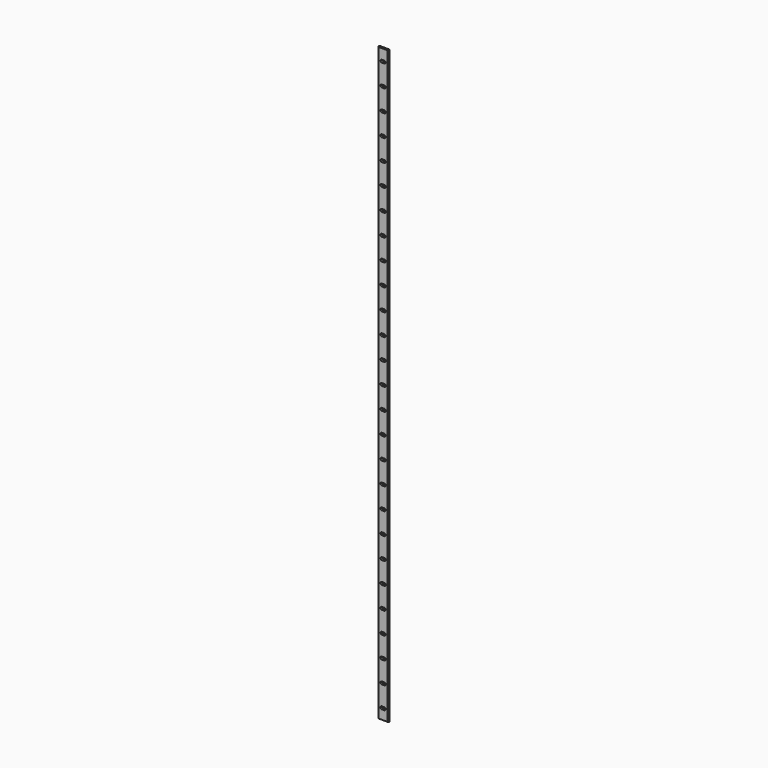
from build123d import *

# Parameters (mm, degrees)
F1_DEPTH = 1350
F2_R     = 0.5
F3_ANGLE = 180
F6_DEPTH = 25


with BuildPart() as f1:
    # F0 (on Top) → F1 (new body)
    with BuildSketch(Plane.XY):
        Polygon((20.122, 0), (0, 0), (0, -2.375), (19.5291, -2.375), (19.5291, -4.75), (20.122, -4.75), (22.497, -2.375), align=None)
    extrude(amount=F1_DEPTH)

    # F2
    f2_edges = [f1.edges().sort_by_distance(p)[0] for p in [
        (20.122, -4.75, 675),
        (22.497, -2.375, 675),
        (20.122, 0, 675),
    ]]
    fillet(f2_edges, radius=F2_R)


with BuildPart() as f3_1:
    # F3: copy of F1
    add(f1.part.rotate(Axis((0, -2.375, 675), (0, 0, -1)), F3_ANGLE))


with BuildPart() as f3_1_1:
    # F4: moved
    add(f3_1.part.moved(Location((19.5291, 0, 0))))


with BuildPart() as f6_tool:
    # F5 (on face) → F6 (new body)
    with BuildSketch(Plane.XZ.offset(4.75)):
        with BuildLine():
            ThreePointArc((6.7392067812, 1320.875), (8.4185023577, 1321.3645510123), (9.5716533906, 1322.6798215254))
            ThreePointArc((9.5716533906, 1322.6798215254), (10.7248044235, 1321.3645510123), (12.4041, 1320.875))
            ThreePointArc((12.4041, 1320.875), (15.5291, 1324), (12.4041, 1327.125))
            Line((12.4041, 1327.125), (6.7392067812, 1327.125))
            ThreePointArc((6.7392067812, 1327.125), (3.6142067812, 1324), (6.7392067812, 1320.875))
        make_face()
        with BuildLine():
            ThreePointArc((12.4041, 1320.875), (10.7248044235, 1321.3645510123), (9.5716533906, 1322.6798215254))
            ThreePointArc((9.5716533906, 1322.6798215254), (8.4185023577, 1321.3645510123), (6.7392067812, 1320.875))
            Line((6.7392067812, 1320.875), (12.4041, 1320.875))
        make_face()
        with BuildLine():
            Line((12.4041, 1277.125), (6.7392067812, 1277.125))
            ThreePointArc((6.7392067812, 1277.125), (3.6142067812, 1274), (6.7392067812, 1270.875))
            ThreePointArc((6.7392067812, 1270.875), (8.4185023577, 1271.3645510123), (9.5716533906, 1272.6798215254))
            ThreePointArc((9.5716533906, 1272.6798215254), (10.7248044235, 1271.3645510123), (12.4041, 1270.875))
            ThreePointArc((12.4041, 1270.875), (15.5291, 1274), (12.4041, 1277.125))
        make_face()
        with BuildLine():
            ThreePointArc((9.5716533906, 1272.6798215254), (8.4185023577, 1271.3645510123), (6.7392067812, 1270.875))
            Line((6.7392067812, 1270.875), (12.4041, 1270.875))
            ThreePointArc((12.4041, 1270.875), (10.7248044235, 1271.3645510123), (9.5716533906, 1272.6798215254))
        make_face()
        with BuildLine():
            Line((12.4041, 1227.125), (6.7392067812, 1227.125))
            ThreePointArc((6.7392067812, 1227.125), (3.6142067812, 1224), (6.7392067812, 1220.875))
            ThreePointArc((6.7392067812, 1220.875), (8.4185023577, 1221.3645510123), (9.5716533906, 1222.6798215254))
            ThreePointArc((9.5716533906, 1222.6798215254), (10.7248044235, 1221.3645510123), (12.4041, 1220.875))
            ThreePointArc((12.4041, 1220.875), (15.5291, 1224), (12.4041, 1227.125))
        make_face()
        with BuildLine():
            ThreePointArc((9.5716533906, 1222.6798215254), (8.4185023577, 1221.3645510123), (6.7392067812, 1220.875))
            Line((6.7392067812, 1220.875), (12.4041, 1220.875))
            ThreePointArc((12.4041, 1220.875), (10.7248044235, 1221.3645510123), (9.5716533906, 1222.6798215254))
        make_face()
        with BuildLine():
            Line((12.4041, 1177.125), (6.7392067812, 1177.125))
            ThreePointArc((6.7392067812, 1177.125), (3.6142067812, 1174), (6.7392067812, 1170.875))
            ThreePointArc((6.7392067812, 1170.875), (8.4185023577, 1171.3645510123), (9.5716533906, 1172.6798215254))
            ThreePointArc((9.5716533906, 1172.6798215254), (10.7248044235, 1171.3645510123), (12.4041, 1170.875))
            ThreePointArc((12.4041, 1170.875), (15.5291, 1174), (12.4041, 1177.125))
        make_face()
        with BuildLine():
            ThreePointArc((9.5716533906, 1172.6798215254), (8.4185023577, 1171.3645510123), (6.7392067812, 1170.875))
            Line((6.7392067812, 1170.875), (12.4041, 1170.875))
            ThreePointArc((12.4041, 1170.875), (10.7248044235, 1171.3645510123), (9.5716533906, 1172.6798215254))
        make_face()
        with BuildLine():
            Line((12.4041, 1127.125), (6.7392067812, 1127.125))
            ThreePointArc((6.7392067812, 1127.125), (3.6142067812, 1124), (6.7392067812, 1120.875))
            ThreePointArc((6.7392067812, 1120.875), (8.4185023577, 1121.3645510123), (9.5716533906, 1122.6798215254))
            ThreePointArc((9.5716533906, 1122.6798215254), (10.7248044235, 1121.3645510123), (12.4041, 1120.875))
            ThreePointArc((12.4041, 1120.875), (15.5291, 1124), (12.4041, 1127.125))
        make_face()
        with BuildLine():
            ThreePointArc((9.5716533906, 1122.6798215254), (8.4185023577, 1121.3645510123), (6.7392067812, 1120.875))
            Line((6.7392067812, 1120.875), (12.4041, 1120.875))
            ThreePointArc((12.4041, 1120.875), (10.7248044235, 1121.3645510123), (9.5716533906, 1122.6798215254))
        make_face()
        with BuildLine():
            Line((12.4041, 1077.125), (6.7392067812, 1077.125))
            ThreePointArc((6.7392067812, 1077.125), (3.6142067812, 1074), (6.7392067812, 1070.875))
            ThreePointArc((6.7392067812, 1070.875), (8.4185023577, 1071.3645510123), (9.5716533906, 1072.6798215254))
            ThreePointArc((9.5716533906, 1072.6798215254), (10.7248044235, 1071.3645510123), (12.4041, 1070.875))
            ThreePointArc((12.4041, 1070.875), (15.5291, 1074), (12.4041, 1077.125))
        make_face()
        with BuildLine():
            ThreePointArc((9.5716533906, 1072.6798215254), (8.4185023577, 1071.3645510123), (6.7392067812, 1070.875))
            Line((6.7392067812, 1070.875), (12.4041, 1070.875))
            ThreePointArc((12.4041, 1070.875), (10.7248044235, 1071.3645510123), (9.5716533906, 1072.6798215254))
        make_face()
        with BuildLine():
            Line((12.4041, 1027.125), (6.7392067812, 1027.125))
            ThreePointArc((6.7392067812, 1027.125), (3.6142067812, 1024), (6.7392067812, 1020.875))
            ThreePointArc((6.7392067812, 1020.875), (8.4185023577, 1021.3645510123), (9.5716533906, 1022.6798215254))
            ThreePointArc((9.5716533906, 1022.6798215254), (10.7248044235, 1021.3645510123), (12.4041, 1020.875))
            ThreePointArc((12.4041, 1020.875), (15.5291, 1024), (12.4041, 1027.125))
        make_face()
        with BuildLine():
            ThreePointArc((9.5716533906, 1022.6798215254), (8.4185023577, 1021.3645510123), (6.7392067812, 1020.875))
            Line((6.7392067812, 1020.875), (12.4041, 1020.875))
            ThreePointArc((12.4041, 1020.875), (10.7248044235, 1021.3645510123), (9.5716533906, 1022.6798215254))
        make_face()
        with BuildLine():
            Line((12.4041, 977.125), (6.7392067812, 977.125))
            ThreePointArc((6.7392067812, 977.125), (3.6142067812, 974), (6.7392067812, 970.875))
            ThreePointArc((6.7392067812, 970.875), (8.4185023577, 971.3645510123), (9.5716533906, 972.6798215254))
            ThreePointArc((9.5716533906, 972.6798215254), (10.7248044235, 971.3645510123), (12.4041, 970.875))
            ThreePointArc((12.4041, 970.875), (15.5291, 974), (12.4041, 977.125))
        make_face()
        with BuildLine():
            ThreePointArc((9.5716533906, 972.6798215254), (8.4185023577, 971.3645510123), (6.7392067812, 970.875))
            Line((6.7392067812, 970.875), (12.4041, 970.875))
            ThreePointArc((12.4041, 970.875), (10.7248044235, 971.3645510123), (9.5716533906, 972.6798215254))
        make_face()
        with BuildLine():
            Line((12.4041, 927.125), (6.7392067812, 927.125))
            ThreePointArc((6.7392067812, 927.125), (3.6142067812, 924), (6.7392067812, 920.875))
            ThreePointArc((6.7392067812, 920.875), (8.4185023577, 921.3645510123), (9.5716533906, 922.6798215254))
            ThreePointArc((9.5716533906, 922.6798215254), (10.7248044235, 921.3645510123), (12.4041, 920.875))
            ThreePointArc((12.4041, 920.875), (15.5291, 924), (12.4041, 927.125))
        make_face()
        with BuildLine():
            ThreePointArc((9.5716533906, 922.6798215254), (8.4185023577, 921.3645510123), (6.7392067812, 920.875))
            Line((6.7392067812, 920.875), (12.4041, 920.875))
            ThreePointArc((12.4041, 920.875), (10.7248044235, 921.3645510123), (9.5716533906, 922.6798215254))
        make_face()
        with BuildLine():
            Line((12.4041, 877.125), (6.7392067812, 877.125))
            ThreePointArc((6.7392067812, 877.125), (3.6142067812, 874), (6.7392067812, 870.875))
            ThreePointArc((6.7392067812, 870.875), (8.4185023577, 871.3645510123), (9.5716533906, 872.6798215254))
            ThreePointArc((9.5716533906, 872.6798215254), (10.7248044235, 871.3645510123), (12.4041, 870.875))
            ThreePointArc((12.4041, 870.875), (15.5291, 874), (12.4041, 877.125))
        make_face()
        with BuildLine():
            ThreePointArc((9.5716533906, 872.6798215254), (8.4185023577, 871.3645510123), (6.7392067812, 870.875))
            Line((6.7392067812, 870.875), (12.4041, 870.875))
            ThreePointArc((12.4041, 870.875), (10.7248044235, 871.3645510123), (9.5716533906, 872.6798215254))
        make_face()
        with BuildLine():
            Line((12.4041, 827.125), (6.7392067812, 827.125))
            ThreePointArc((6.7392067812, 827.125), (3.6142067812, 824), (6.7392067812, 820.875))
            ThreePointArc((6.7392067812, 820.875), (8.4185023577, 821.3645510123), (9.5716533906, 822.6798215254))
            ThreePointArc((9.5716533906, 822.6798215254), (10.7248044235, 821.3645510123), (12.4041, 820.875))
            ThreePointArc((12.4041, 820.875), (15.5291, 824), (12.4041, 827.125))
        make_face()
        with BuildLine():
            ThreePointArc((9.5716533906, 822.6798215254), (8.4185023577, 821.3645510123), (6.7392067812, 820.875))
            Line((6.7392067812, 820.875), (12.4041, 820.875))
            ThreePointArc((12.4041, 820.875), (10.7248044235, 821.3645510123), (9.5716533906, 822.6798215254))
        make_face()
        with BuildLine():
            Line((12.4041, 777.125), (6.7392067812, 777.125))
            ThreePointArc((6.7392067812, 777.125), (3.6142067812, 774), (6.7392067812, 770.875))
            ThreePointArc((6.7392067812, 770.875), (8.4185023577, 771.3645510123), (9.5716533906, 772.6798215254))
            ThreePointArc((9.5716533906, 772.6798215254), (10.7248044235, 771.3645510123), (12.4041, 770.875))
            ThreePointArc((12.4041, 770.875), (15.5291, 774), (12.4041, 777.125))
        make_face()
        with BuildLine():
            ThreePointArc((9.5716533906, 772.6798215254), (8.4185023577, 771.3645510123), (6.7392067812, 770.875))
            Line((6.7392067812, 770.875), (12.4041, 770.875))
            ThreePointArc((12.4041, 770.875), (10.7248044235, 771.3645510123), (9.5716533906, 772.6798215254))
        make_face()
        with BuildLine():
            Line((12.4041, 727.125), (6.7392067812, 727.125))
            ThreePointArc((6.7392067812, 727.125), (3.6142067812, 724), (6.7392067812, 720.875))
            ThreePointArc((6.7392067812, 720.875), (8.4185023577, 721.3645510123), (9.5716533906, 722.6798215254))
            ThreePointArc((9.5716533906, 722.6798215254), (10.7248044235, 721.3645510123), (12.4041, 720.875))
            ThreePointArc((12.4041, 720.875), (15.5291, 724), (12.4041, 727.125))
        make_face()
        with BuildLine():
            ThreePointArc((9.5716533906, 722.6798215254), (8.4185023577, 721.3645510123), (6.7392067812, 720.875))
            Line((6.7392067812, 720.875), (12.4041, 720.875))
            ThreePointArc((12.4041, 720.875), (10.7248044235, 721.3645510123), (9.5716533906, 722.6798215254))
        make_face()
        with BuildLine():
            Line((12.4041, 677.125), (6.7392067812, 677.125))
            ThreePointArc((6.7392067812, 677.125), (3.6142067812, 674), (6.7392067812, 670.875))
            ThreePointArc((6.7392067812, 670.875), (8.4185023577, 671.3645510123), (9.5716533906, 672.6798215254))
            ThreePointArc((9.5716533906, 672.6798215254), (10.7248044235, 671.3645510123), (12.4041, 670.875))
            ThreePointArc((12.4041, 670.875), (15.5291, 674), (12.4041, 677.125))
        make_face()
        with BuildLine():
            ThreePointArc((9.5716533906, 672.6798215254), (8.4185023577, 671.3645510123), (6.7392067812, 670.875))
            Line((6.7392067812, 670.875), (12.4041, 670.875))
            ThreePointArc((12.4041, 670.875), (10.7248044235, 671.3645510123), (9.5716533906, 672.6798215254))
        make_face()
        with BuildLine():
            Line((12.4041, 627.125), (6.7392067812, 627.125))
            ThreePointArc((6.7392067812, 627.125), (3.6142067812, 624), (6.7392067812, 620.875))
            ThreePointArc((6.7392067812, 620.875), (8.4185023577, 621.3645510123), (9.5716533906, 622.6798215254))
            ThreePointArc((9.5716533906, 622.6798215254), (10.7248044235, 621.3645510123), (12.4041, 620.875))
            ThreePointArc((12.4041, 620.875), (15.5291, 624), (12.4041, 627.125))
        make_face()
        with BuildLine():
            ThreePointArc((9.5716533906, 622.6798215254), (8.4185023577, 621.3645510123), (6.7392067812, 620.875))
            Line((6.7392067812, 620.875), (12.4041, 620.875))
            ThreePointArc((12.4041, 620.875), (10.7248044235, 621.3645510123), (9.5716533906, 622.6798215254))
        make_face()
        with BuildLine():
            Line((12.4041, 577.125), (6.7392067812, 577.125))
            ThreePointArc((6.7392067812, 577.125), (3.6142067812, 574), (6.7392067812, 570.875))
            ThreePointArc((6.7392067812, 570.875), (8.4185023577, 571.3645510123), (9.5716533906, 572.6798215254))
            ThreePointArc((9.5716533906, 572.6798215254), (10.7248044235, 571.3645510123), (12.4041, 570.875))
            ThreePointArc((12.4041, 570.875), (15.5291, 574), (12.4041, 577.125))
        make_face()
        with BuildLine():
            ThreePointArc((9.5716533906, 572.6798215254), (8.4185023577, 571.3645510123), (6.7392067812, 570.875))
            Line((6.7392067812, 570.875), (12.4041, 570.875))
            ThreePointArc((12.4041, 570.875), (10.7248044235, 571.3645510123), (9.5716533906, 572.6798215254))
        make_face()
        with BuildLine():
            Line((12.4041, 527.125), (6.7392067812, 527.125))
            ThreePointArc((6.7392067812, 527.125), (3.6142067812, 524), (6.7392067812, 520.875))
            ThreePointArc((6.7392067812, 520.875), (8.4185023577, 521.3645510123), (9.5716533906, 522.6798215254))
            ThreePointArc((9.5716533906, 522.6798215254), (10.7248044235, 521.3645510123), (12.4041, 520.875))
            ThreePointArc((12.4041, 520.875), (15.5291, 524), (12.4041, 527.125))
        make_face()
        with BuildLine():
            ThreePointArc((9.5716533906, 522.6798215254), (8.4185023577, 521.3645510123), (6.7392067812, 520.875))
            Line((6.7392067812, 520.875), (12.4041, 520.875))
            ThreePointArc((12.4041, 520.875), (10.7248044235, 521.3645510123), (9.5716533906, 522.6798215254))
        make_face()
        with BuildLine():
            Line((12.4041, 477.125), (6.7392067812, 477.125))
            ThreePointArc((6.7392067812, 477.125), (3.6142067812, 474), (6.7392067812, 470.875))
            ThreePointArc((6.7392067812, 470.875), (8.4185023577, 471.3645510123), (9.5716533906, 472.6798215254))
            ThreePointArc((9.5716533906, 472.6798215254), (10.7248044235, 471.3645510123), (12.4041, 470.875))
            ThreePointArc((12.4041, 470.875), (15.5291, 474), (12.4041, 477.125))
        make_face()
        with BuildLine():
            ThreePointArc((9.5716533906, 472.6798215254), (8.4185023577, 471.3645510123), (6.7392067812, 470.875))
            Line((6.7392067812, 470.875), (12.4041, 470.875))
            ThreePointArc((12.4041, 470.875), (10.7248044235, 471.3645510123), (9.5716533906, 472.6798215254))
        make_face()
        with BuildLine():
            Line((12.4041, 427.125), (6.7392067812, 427.125))
            ThreePointArc((6.7392067812, 427.125), (3.6142067812, 424), (6.7392067812, 420.875))
            ThreePointArc((6.7392067812, 420.875), (8.4185023577, 421.3645510123), (9.5716533906, 422.6798215254))
            ThreePointArc((9.5716533906, 422.6798215254), (10.7248044235, 421.3645510123), (12.4041, 420.875))
            ThreePointArc((12.4041, 420.875), (15.5291, 424), (12.4041, 427.125))
        make_face()
        with BuildLine():
            ThreePointArc((9.5716533906, 422.6798215254), (8.4185023577, 421.3645510123), (6.7392067812, 420.875))
            Line((6.7392067812, 420.875), (12.4041, 420.875))
            ThreePointArc((12.4041, 420.875), (10.7248044235, 421.3645510123), (9.5716533906, 422.6798215254))
        make_face()
        with BuildLine():
            Line((12.4041, 377.125), (6.7392067812, 377.125))
            ThreePointArc((6.7392067812, 377.125), (3.6142067812, 374), (6.7392067812, 370.875))
            ThreePointArc((6.7392067812, 370.875), (8.4185023577, 371.3645510123), (9.5716533906, 372.6798215254))
            ThreePointArc((9.5716533906, 372.6798215254), (10.7248044235, 371.3645510123), (12.4041, 370.875))
            ThreePointArc((12.4041, 370.875), (15.5291, 374), (12.4041, 377.125))
        make_face()
        with BuildLine():
            ThreePointArc((9.5716533906, 372.6798215254), (8.4185023577, 371.3645510123), (6.7392067812, 370.875))
            Line((6.7392067812, 370.875), (12.4041, 370.875))
            ThreePointArc((12.4041, 370.875), (10.7248044235, 371.3645510123), (9.5716533906, 372.6798215254))
        make_face()
        with BuildLine():
            Line((12.4041, 327.125), (6.7392067812, 327.125))
            ThreePointArc((6.7392067812, 327.125), (3.6142067812, 324), (6.7392067812, 320.875))
            ThreePointArc((6.7392067812, 320.875), (8.4185023577, 321.3645510123), (9.5716533906, 322.6798215254))
            ThreePointArc((9.5716533906, 322.6798215254), (10.7248044235, 321.3645510123), (12.4041, 320.875))
            ThreePointArc((12.4041, 320.875), (15.5291, 324), (12.4041, 327.125))
        make_face()
        with BuildLine():
            ThreePointArc((9.5716533906, 322.6798215254), (8.4185023577, 321.3645510123), (6.7392067812, 320.875))
            Line((6.7392067812, 320.875), (12.4041, 320.875))
            ThreePointArc((12.4041, 320.875), (10.7248044235, 321.3645510123), (9.5716533906, 322.6798215254))
        make_face()
        with BuildLine():
            Line((12.4041, 277.125), (6.7392067812, 277.125))
            ThreePointArc((6.7392067812, 277.125), (3.6142067812, 274), (6.7392067812, 270.875))
            ThreePointArc((6.7392067812, 270.875), (8.4185023577, 271.3645510123), (9.5716533906, 272.6798215254))
            ThreePointArc((9.5716533906, 272.6798215254), (10.7248044235, 271.3645510123), (12.4041, 270.875))
            ThreePointArc((12.4041, 270.875), (15.5291, 274), (12.4041, 277.125))
        make_face()
        with BuildLine():
            ThreePointArc((9.5716533906, 272.6798215254), (8.4185023577, 271.3645510123), (6.7392067812, 270.875))
            Line((6.7392067812, 270.875), (12.4041, 270.875))
            ThreePointArc((12.4041, 270.875), (10.7248044235, 271.3645510123), (9.5716533906, 272.6798215254))
        make_face()
        with BuildLine():
            Line((12.4041, 227.125), (6.7392067812, 227.125))
            ThreePointArc((6.7392067812, 227.125), (3.6142067812, 224), (6.7392067812, 220.875))
            ThreePointArc((6.7392067812, 220.875), (8.4185023577, 221.3645510123), (9.5716533906, 222.6798215254))
            ThreePointArc((9.5716533906, 222.6798215254), (10.7248044235, 221.3645510123), (12.4041, 220.875))
            ThreePointArc((12.4041, 220.875), (15.5291, 224), (12.4041, 227.125))
        make_face()
        with BuildLine():
            ThreePointArc((9.5716533906, 222.6798215254), (8.4185023577, 221.3645510123), (6.7392067812, 220.875))
            Line((6.7392067812, 220.875), (12.4041, 220.875))
            ThreePointArc((12.4041, 220.875), (10.7248044235, 221.3645510123), (9.5716533906, 222.6798215254))
        make_face()
        with BuildLine():
            Line((12.4041, 177.125), (6.7392067812, 177.125))
            ThreePointArc((6.7392067812, 177.125), (3.6142067812, 174), (6.7392067812, 170.875))
            ThreePointArc((6.7392067812, 170.875), (8.4185023577, 171.3645510123), (9.5716533906, 172.6798215254))
            ThreePointArc((9.5716533906, 172.6798215254), (10.7248044235, 171.3645510123), (12.4041, 170.875))
            ThreePointArc((12.4041, 170.875), (15.5291, 174), (12.4041, 177.125))
        make_face()
        with BuildLine():
            ThreePointArc((9.5716533906, 172.6798215254), (8.4185023577, 171.3645510123), (6.7392067812, 170.875))
            Line((6.7392067812, 170.875), (12.4041, 170.875))
            ThreePointArc((12.4041, 170.875), (10.7248044235, 171.3645510123), (9.5716533906, 172.6798215254))
        make_face()
        with BuildLine():
            Line((12.4041, 127.125), (6.7392067812, 127.125))
            ThreePointArc((6.7392067812, 127.125), (3.6142067812, 124), (6.7392067812, 120.875))
            ThreePointArc((6.7392067812, 120.875), (8.4185023577, 121.3645510123), (9.5716533906, 122.6798215254))
            ThreePointArc((9.5716533906, 122.6798215254), (10.7248044235, 121.3645510123), (12.4041, 120.875))
            ThreePointArc((12.4041, 120.875), (15.5291, 124), (12.4041, 127.125))
        make_face()
        with BuildLine():
            ThreePointArc((9.5716533906, 122.6798215254), (8.4185023577, 121.3645510123), (6.7392067812, 120.875))
            Line((6.7392067812, 120.875), (12.4041, 120.875))
            ThreePointArc((12.4041, 120.875), (10.7248044235, 121.3645510123), (9.5716533906, 122.6798215254))
        make_face()
        with BuildLine():
            Line((12.4041, 77.125), (6.7392067812, 77.125))
            ThreePointArc((6.7392067812, 77.125), (3.6142067812, 74), (6.7392067812, 70.875))
            ThreePointArc((6.7392067812, 70.875), (8.4185023577, 71.3645510123), (9.5716533906, 72.6798215254))
            ThreePointArc((9.5716533906, 72.6798215254), (10.7248044235, 71.3645510123), (12.4041, 70.875))
            ThreePointArc((12.4041, 70.875), (15.5291, 74), (12.4041, 77.125))
        make_face()
        with BuildLine():
            ThreePointArc((9.5716533906, 72.6798215254), (8.4185023577, 71.3645510123), (6.7392067812, 70.875))
            Line((6.7392067812, 70.875), (12.4041, 70.875))
            ThreePointArc((12.4041, 70.875), (10.7248044235, 71.3645510123), (9.5716533906, 72.6798215254))
        make_face()
        with BuildLine():
            Line((12.4041, 27.125), (6.7392067812, 27.125))
            ThreePointArc((6.7392067812, 27.125), (3.6142067812, 24), (6.7392067812, 20.875))
            ThreePointArc((6.7392067812, 20.875), (8.4185023577, 21.3645510123), (9.5716533906, 22.6798215254))
            ThreePointArc((9.5716533906, 22.6798215254), (10.7248044235, 21.3645510123), (12.4041, 20.875))
            ThreePointArc((12.4041, 20.875), (15.5291, 24), (12.4041, 27.125))
        make_face()
        with BuildLine():
            ThreePointArc((9.5716533906, 22.6798215254), (8.4185023577, 21.3645510123), (6.7392067812, 20.875))
            Line((6.7392067812, 20.875), (12.4041, 20.875))
            ThreePointArc((12.4041, 20.875), (10.7248044235, 21.3645510123), (9.5716533906, 22.6798215254))
        make_face()
        with BuildLine():
            Line((12.4041, -22.875), (6.7392067812, -22.875))
            ThreePointArc((6.7392067812, -22.875), (3.6142067812, -26), (6.7392067812, -29.125))
            ThreePointArc((6.7392067812, -29.125), (8.4185023577, -28.6354489877), (9.5716533906, -27.3201784746))
            ThreePointArc((9.5716533906, -27.3201784746), (10.7248044235, -28.6354489877), (12.4041, -29.125))
            ThreePointArc((12.4041, -29.125), (15.5291, -26), (12.4041, -22.875))
        make_face()
        with BuildLine():
            ThreePointArc((9.5716533906, -27.3201784746), (8.4185023577, -28.6354489877), (6.7392067812, -29.125))
            Line((6.7392067812, -29.125), (12.4041, -29.125))
            ThreePointArc((12.4041, -29.125), (10.7248044235, -28.6354489877), (9.5716533906, -27.3201784746))
        make_face()
        with BuildLine():
            Line((12.4041, -72.875), (6.7392067812, -72.875))
            ThreePointArc((6.7392067812, -72.875), (3.6142067812, -76), (6.7392067812, -79.125))
            ThreePointArc((6.7392067812, -79.125), (8.4185023577, -78.6354489877), (9.5716533906, -77.3201784746))
            ThreePointArc((9.5716533906, -77.3201784746), (10.7248044235, -78.6354489877), (12.4041, -79.125))
            ThreePointArc((12.4041, -79.125), (15.5291, -76), (12.4041, -72.875))
        make_face()
        with BuildLine():
            ThreePointArc((9.5716533906, -77.3201784746), (8.4185023577, -78.6354489877), (6.7392067812, -79.125))
            Line((6.7392067812, -79.125), (12.4041, -79.125))
            ThreePointArc((12.4041, -79.125), (10.7248044235, -78.6354489877), (9.5716533906, -77.3201784746))
        make_face()
        with BuildLine():
            Line((12.4041, -122.875), (6.7392067812, -122.875))
            ThreePointArc((6.7392067812, -122.875), (3.6142067812, -126), (6.7392067812, -129.125))
            ThreePointArc((6.7392067812, -129.125), (8.4185023577, -128.6354489877), (9.5716533906, -127.3201784746))
            ThreePointArc((9.5716533906, -127.3201784746), (10.7248044235, -128.6354489877), (12.4041, -129.125))
            ThreePointArc((12.4041, -129.125), (15.5291, -126), (12.4041, -122.875))
        make_face()
        with BuildLine():
            ThreePointArc((9.5716533906, -127.3201784746), (8.4185023577, -128.6354489877), (6.7392067812, -129.125))
            Line((6.7392067812, -129.125), (12.4041, -129.125))
            ThreePointArc((12.4041, -129.125), (10.7248044235, -128.6354489877), (9.5716533906, -127.3201784746))
        make_face()
    extrude(amount=-F6_DEPTH)


with BuildPart() as f1_1:
    add(f1.part)

    # F6: cut by f6_tool
    add(f6_tool.part, mode=Mode.SUBTRACT)


with BuildPart() as f3_1_2:
    add(f3_1_1.part)

    # F6: cut by f6_tool
    add(f6_tool.part, mode=Mode.SUBTRACT)


solid = Compound([f1_1.part, f3_1_2.part])
